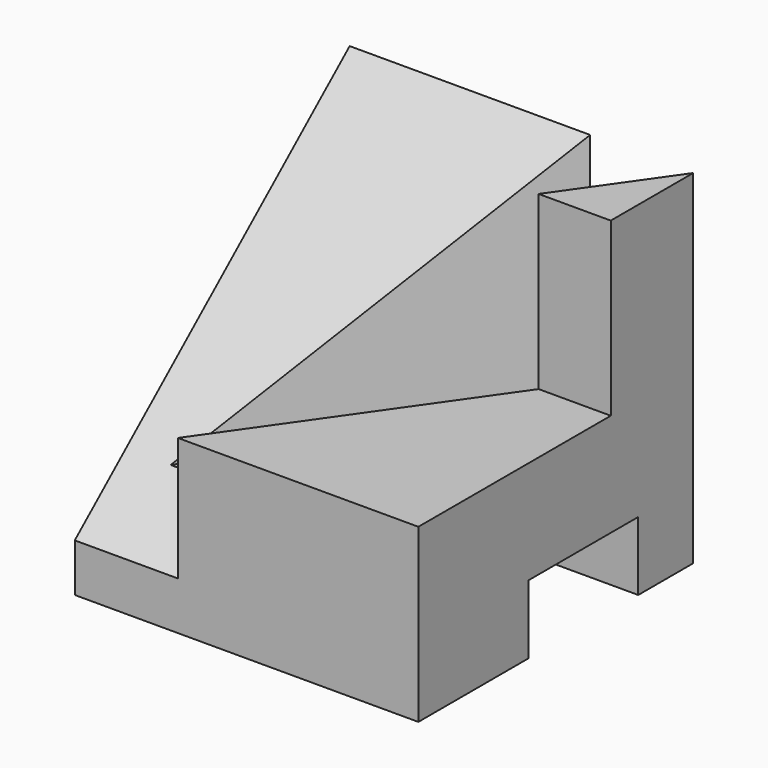
from build123d import *

# Parameters (mm, degrees)
F0_W      = 50
F0_H      = 50
F1_DEPTH  = 50
F5_W      = 20
F5_H      = 10
F6_DEPTH  = 30
F8_DEPTH  = 35
F10_DEPTH = 25
F12_REACH = 115.9479483752


with BuildPart() as f1:
    # F0 (on Top) → F1 (new body)
    with BuildSketch(Plane.XY):
        with Locations((25, 25)):
            Rectangle(F0_W, F0_H)
    extrude(amount=F1_DEPTH)

    # F5 (on face) → F6 (cut)
    with BuildSketch(Plane.YZ.offset(50)):
        with Locations((30, 5)):
            Rectangle(F5_W, F5_H)
    extrude(amount=-F6_DEPTH, mode=Mode.SUBTRACT)

    # F7 (on face) → F8 (cut)
    with BuildSketch(Plane.XY.offset(50)):
        Polygon((15, 0), (50, 50), (35, 50), (0, 0), align=None)
    extrude(amount=-F8_DEPTH, mode=Mode.SUBTRACT)

    # F9 (on face) → F10 (cut)
    with BuildSketch(Plane.XY.offset(50)):
        Polygon((50, 35), (39.5, 35), (15, 0), (50, 0), align=None)
    extrude(amount=-F10_DEPTH, mode=Mode.SUBTRACT)

    f12_end = Plane(origin=(37.75, 32.5, 27.5), x_dir=(-0.5734623444, -0.8192319205, 0), z_dir=(-0.8192319205, 0.5734623444, 0))
    # F11 (on face) → F12 (cut, up to a plane its end follows)
    with BuildSketch(Plane(origin=(0, 0, 0), x_dir=(0, -1, 0), z_dir=(-1, 0, 0))):
        Polygon((0, 7), (0, 50), (-50, 50), align=None)
    f12_long = extrude(amount=-F12_REACH, mode=Mode.PRIVATE)
    add(split(f12_long, bisect_by=f12_end, keep=Keep.TOP, mode=Mode.PRIVATE), mode=Mode.SUBTRACT)


solid = f1.part
